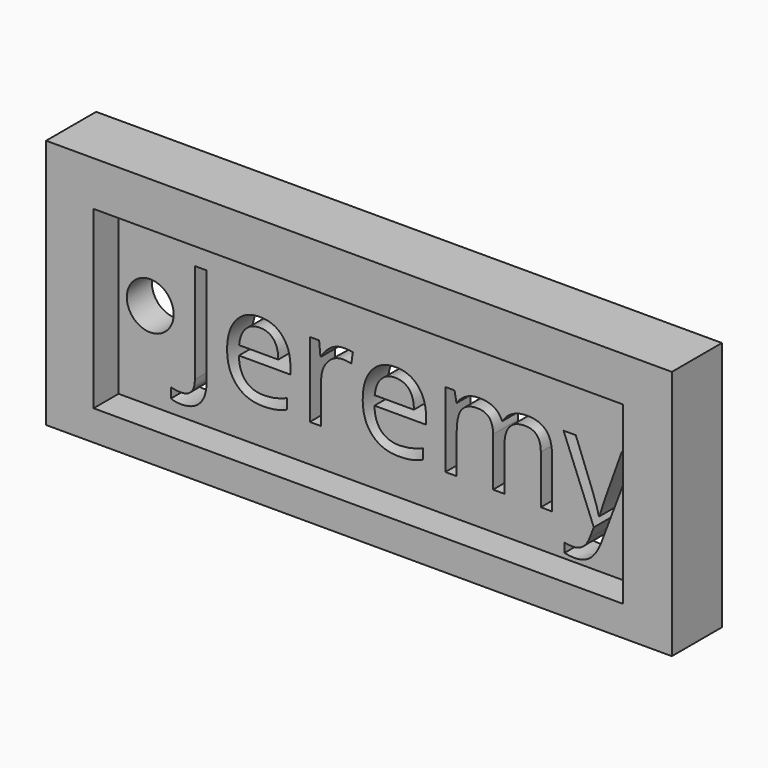
from build123d import *

# Parameters (mm, degrees)
F0_W          = 63.5
F0_H          = 25.4
F0_W_2        = 53.7293371744
F0_H_2        = 17.8124450613
F1_DEPTH      = 6.35
F2_DEPTH      = 3.175
F3_R          = 2.376766617
F4_DEPTH      = 3.175
F5_TEXT_SIZE  = 14.1948008806
F6_DEPTH      = 2.5
F6_DEPTH_BACK = 25.4


# Not quite as in the source:
# - Text() gives the source's letters only with a copy of the font that has no kerning and outlines rounded to 1/6400 em; it was checked with that copy


with BuildPart() as f1:
    # F0 (on Front) → F1 (new body)
    with BuildSketch(Plane.XZ):
        with Locations((31.75, 12.7)):
            Rectangle(F0_W, F0_H)
        with Locations((31.6827909555, 11.9722991949)):
            Rectangle(F0_W_2, F0_H_2, mode=Mode.SUBTRACT)
    extrude(amount=F1_DEPTH)

    # F0 (on Front) → F2 (join)
    with BuildSketch(Plane.XZ):
        with Locations((31.6827909555, 11.9722991949)):
            Rectangle(F0_W_2, F0_H_2)
    extrude(amount=F2_DEPTH)

    # F3 (on face) → F4 (cut)
    with BuildSketch(Plane.XZ.offset(3.175)):
        with Locations((8.0302022398, 11.9722991949)):
            Circle(F3_R)
    extrude(amount=-F4_DEPTH, mode=Mode.SUBTRACT)

    # F5 (on face) → F6 (cut, two sides)
    with BuildSketch(Plane.XZ.offset(3.175)) as f6_sk:
        with Locations((11.2422797829, 6.8621709943)):
            Text('Jeremy', F5_TEXT_SIZE, font='Open Sans', text_align=(TextAlign.LEFT, TextAlign.BOTTOM))
    extrude(amount=F6_DEPTH, mode=Mode.SUBTRACT)
    extrude(f6_sk.sketch, amount=-F6_DEPTH_BACK, mode=Mode.SUBTRACT)


solid = f1.part
